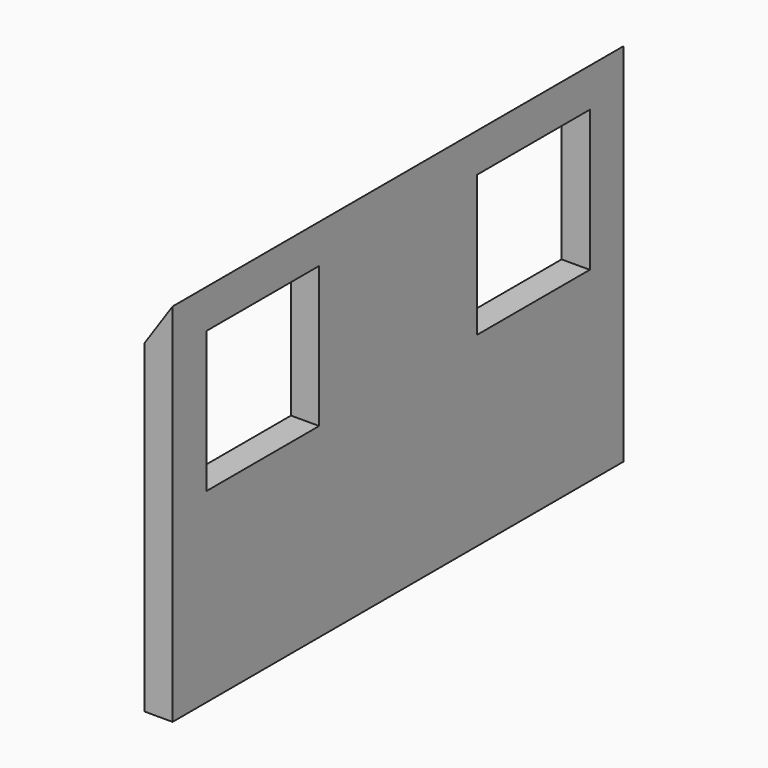
from build123d import *

# Parameters (mm, degrees)
F0_W        = 40
F0_H        = 26.199
F0_W_2      = 10
F0_H_2      = 10
F1_DEPTH    = 2
F2_T1_DEPTH = 56.5285930149


# Not quite as in the source:
# - a fillet or chamfer that OpenCascade refuses, or shapes differently, is made with other operations: its cross-section is extruded or revolved along the edge and cut away or added


with BuildPart() as f1:
    # F0 (on Right) → F1 (new body)
    with BuildSketch(Plane.YZ):
        Rectangle(F0_W, F0_H)
        with Locations((-12, 5.0995)):
            Rectangle(F0_W_2, F0_H_2, mode=Mode.SUBTRACT)
        with Locations((12, 5.0995)):
            Rectangle(F0_W_2, F0_H_2, mode=Mode.SUBTRACT)
    extrude(amount=F1_DEPTH)

    # F2: chamfer of 2.16713 x 3.199 on 1 edges, made by hand

    # F2_s2 → F2_t1 (cut)
    with BuildSketch(Plane.XZ.offset(-28.2642965075)):
        Polygon((2.16713, 13.0995), (0, 9.9005), (0, 13.0995), align=None)
    extrude(amount=F2_T1_DEPTH, mode=Mode.SUBTRACT)


solid = f1.part
